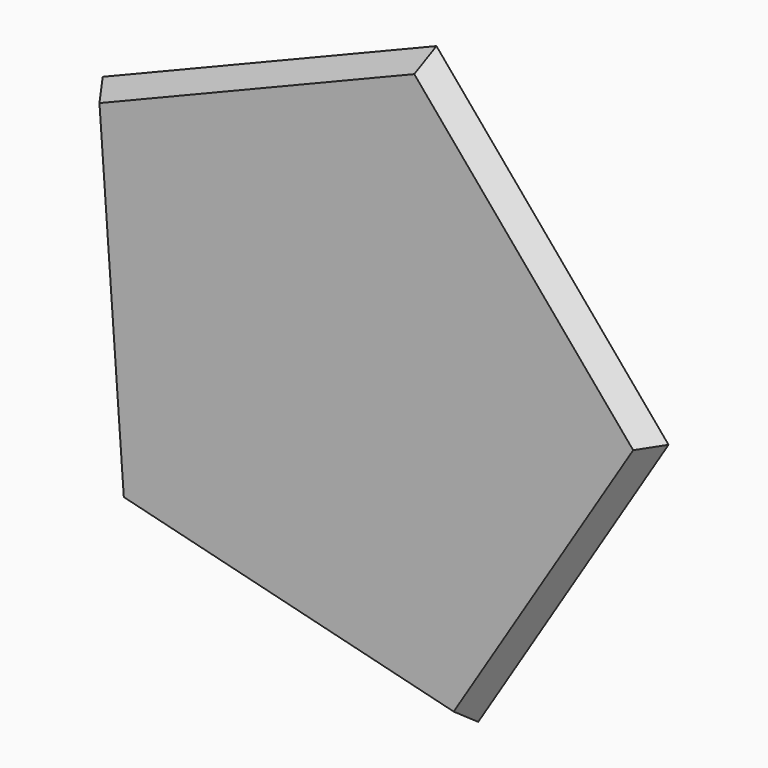
from build123d import *

# Parameters (mm, degrees)
F1_DEPTH = 5
F2_SIZE2 = 3.124337
F2_SIZE  = 4.99999


# Not quite as in the source:
# - a fillet or chamfer is up to 0.001 mm smaller than in the source, because OpenCascade refuses the exact size


with BuildPart() as f1:
    # F0 (on Front) → F1 (new body)
    with BuildSketch(Plane.XZ):
        Polygon((-57.7801036188, 35.9519558773), (-52.0473758656, -43.8423787117), (25.6130563086, -63.0480360688), (67.8771152201, 4.8765494973), (16.3373079557, 66.061909406), align=None)
    extrude(amount=F1_DEPTH)

    # F2 (size 5 and 3.1243467595 in the source; OpenCascade refuses exactly that, so slightly less here)
    f2_edges = [f1.edges().sort_by_distance(p)[0] for p in [
        (-54.91374, -5, -3.945211),
        (-20.721398, -5, 51.006933),
        (42.107212, -5, 35.469229),
        (46.745086, -5, -29.085743),
        (-13.21716, -5, -53.445207),
    ]]
    chamfer(f2_edges, length=F2_SIZE, length2=F2_SIZE2)


solid = f1.part
